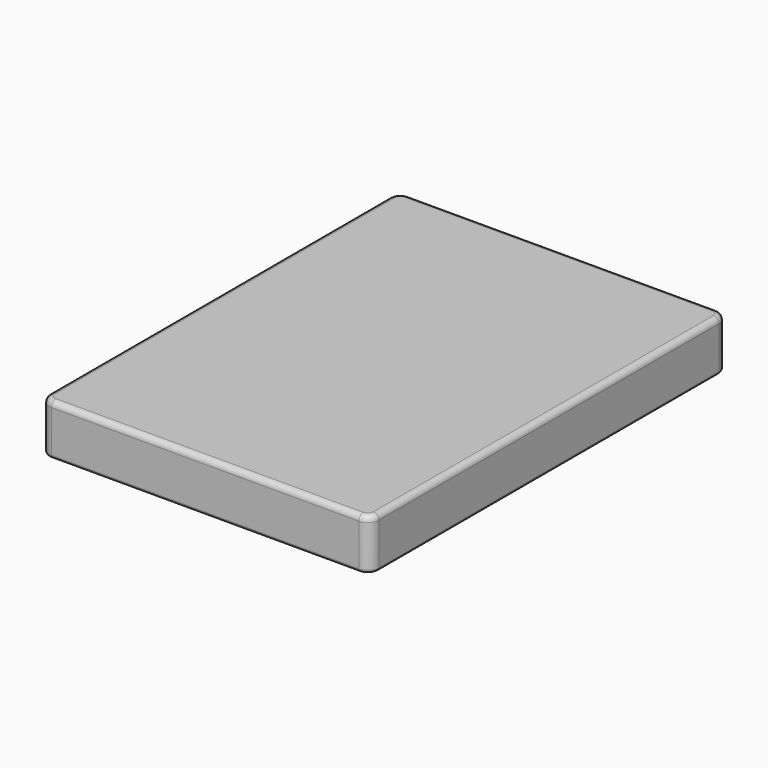
from build123d import *

# Parameters (mm, degrees)
F0_W         = 1498.6
F0_H         = 2032
F1_DEPTH     = 228.6
F2_R         = 25.4
F3_T1_DEPTH  = 355.6
F3_T4_ANGLE  = 90
F3_T6_ANGLE  = 90
F3_T8_ANGLE  = 90
F3_T10_ANGLE = 90
F4_R         = 12.7


# Not quite as in the source:
# - a fillet or chamfer that OpenCascade refuses, or shapes differently, is made with other operations: its cross-section is extruded or revolved along the edge and cut away or added


with BuildPart() as f1:
    # F0 (on Top) → F1 (new body)
    with BuildSketch(Plane.XY):
        Rectangle(F0_W, F0_H)
    extrude(amount=F1_DEPTH)

    # F2
    f2_edges = [f1.edges().sort_by_distance(p)[0] for p in [
        (-749.3, 0, 228.6),
        (0, -1016, 228.6),
        (749.3, 0, 228.6),
        (0, 1016, 228.6),
    ]]
    fillet(f2_edges, radius=F2_R)

    # F3: fillet of radius 50.8 on 4 edges, made by hand

    # F3_s2 → F3_t1 (cut)
    with BuildSketch(Plane.XY.offset(-127)):
        with BuildLine():
            ThreePointArc((-698.5, -1016), (-734.4210244843, -1001.1210244843), (-749.3, -965.2))
            Line((-749.3, -965.2), (-749.3, -1016))
            Line((-749.3, -1016), (-698.5, -1016))
        make_face()
        with BuildLine():
            ThreePointArc((749.3, -965.2), (734.4210244843, -1001.1210244843), (698.5, -1016))
            Line((698.5, -1016), (749.3, -1016))
            Line((749.3, -1016), (749.3, -965.2))
        make_face()
        with BuildLine():
            ThreePointArc((-698.5, 1016), (-734.4210244843, 1001.1210244843), (-749.3, 965.2))
            Line((-749.3, 965.2), (-749.3, 1016))
            Line((-749.3, 1016), (-698.5, 1016))
        make_face()
        with BuildLine():
            ThreePointArc((749.3, 965.2), (734.4210244843, 1001.1210244843), (698.5, 1016))
            Line((698.5, 1016), (749.3, 1016))
            Line((749.3, 1016), (749.3, 965.2))
        make_face()
    extrude(amount=F3_T1_DEPTH, mode=Mode.SUBTRACT)

    # F3_s3 → F3_t4 (revolve, cut)
    with BuildSketch(Plane.XZ.offset(-965.2)):
        with BuildLine():
            ThreePointArc((723.9, 228.6), (741.8605122421, 221.1605122421), (749.3, 203.2))
            Line((749.3, 203.2), (749.3, 228.6))
            Line((749.3, 228.6), (723.9, 228.6))
        make_face()
    revolve(axis=Axis((698.5, 965.2, 228.6), (0, 0, 1)), revolution_arc=F3_T4_ANGLE, mode=Mode.SUBTRACT)

    # F3_s5 → F3_t6 (revolve, cut)
    with BuildSketch(Plane.YZ.offset(-698.5)):
        with BuildLine():
            ThreePointArc((990.6, 228.6), (1008.5605122421, 221.1605122421), (1016, 203.2))
            Line((1016, 203.2), (1016, 228.6))
            Line((1016, 228.6), (990.6, 228.6))
        make_face()
    revolve(axis=Axis((-698.5, 965.2, 228.6), (0, 0, 1)), revolution_arc=F3_T6_ANGLE, mode=Mode.SUBTRACT)

    # F3_s7 → F3_t8 (revolve, cut)
    with BuildSketch(Plane.YZ.offset(698.5)):
        with BuildLine():
            ThreePointArc((-990.6, 228.6), (-1008.5605122421, 221.1605122421), (-1016, 203.2))
            Line((-1016, 203.2), (-1016, 228.6))
            Line((-1016, 228.6), (-990.6, 228.6))
        make_face()
    revolve(axis=Axis((698.5, -965.2, 228.6), (0, 0, 1)), revolution_arc=F3_T8_ANGLE, mode=Mode.SUBTRACT)

    # F3_s9 → F3_t10 (revolve, cut)
    with BuildSketch(Plane.XZ.offset(965.2)):
        with BuildLine():
            ThreePointArc((-723.9, 228.6), (-741.8605122421, 221.1605122421), (-749.3, 203.2))
            Line((-749.3, 203.2), (-749.3, 228.6))
            Line((-749.3, 228.6), (-723.9, 228.6))
        make_face()
    revolve(axis=Axis((-698.5, -965.2, 228.6), (0, 0, 1)), revolution_arc=F3_T10_ANGLE, mode=Mode.SUBTRACT)

    # F4
    f4_edges = [f1.edges().sort_by_distance(p)[0] for p in [
        (0, 1016, 0),
        (-749.3, 0, 0),
        (0, -1016, 0),
    ]]
    fillet(f4_edges, radius=F4_R)


solid = f1.part
